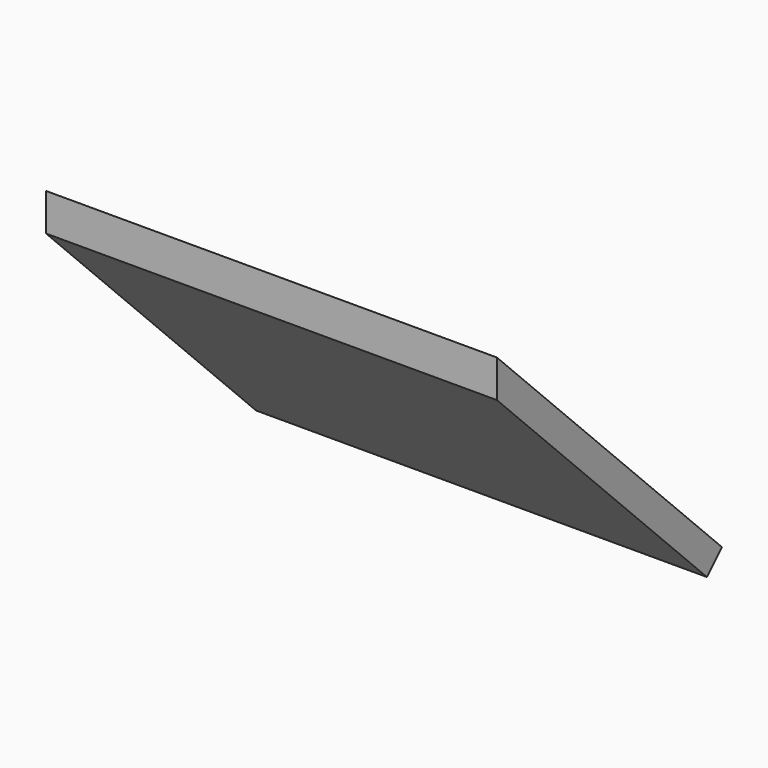
from build123d import *

# Parameters (mm, degrees)
F1_W     = 170
F1_H     = 150
F2_DEPTH = 10
F3_SIZE  = 9.99999


# Not quite as in the source:
# - a fillet or chamfer is up to 0.001 mm smaller than in the source, because OpenCascade refuses the exact size


with BuildPart() as f2:
    # F1 (on face) → F2 (new body)
    with BuildSketch(Plane(origin=(0, 0, 0), x_dir=(-1, 0, 0), z_dir=(0, 0.7071067812, 0.7071067812))):
        Rectangle(F1_W, F1_H)
    extrude(amount=F2_DEPTH)

    # F3 (size 10 in the source; OpenCascade refuses exactly that, so slightly less here)
    f3_edges = [f2.edges().sort_by_distance(p)[0] for p in [
        (0, -53.033009, 53.033009),
    ]]
    chamfer(f3_edges, length=F3_SIZE)


solid = f2.part
